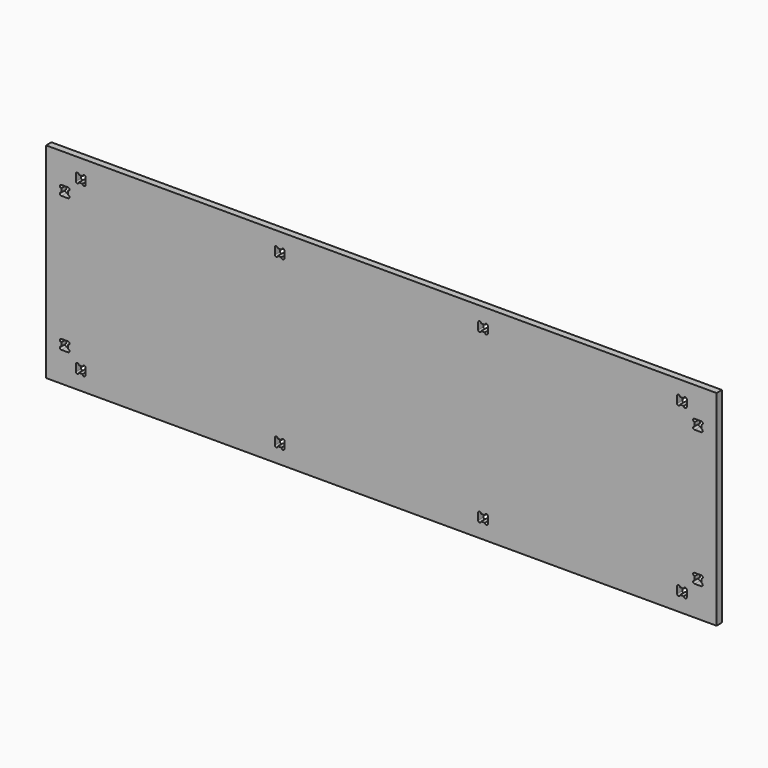
from build123d import *

# Parameters (mm, degrees)
F0_W     = 1800
F0_H     = 550
F1_DEPTH = 18


# Not quite as in the source:
# - ends of sketch curves that miss each other by under 0.0002 mm in the source are joined


with BuildPart() as f1:
    # F0 (on Front) → F1 (new body)
    with BuildSketch(Plane.XZ):
        Rectangle(F0_W, F0_H)
        with BuildLine():
            ThreePointArc((-812.0013296917, -234), (-816.0528989013, -237.9996675633), (-820, -233.8968701525))
            Line((-820, -233.8968701525), (-820, -216.0408403343))
            ThreePointArc((-820, -216.0408403343), (-816.0206289303, -212.0000521246), (-812.000208497, -216))
            Line((-812.000208497, -216), (-801.9986086037, -216))
            ThreePointArc((-801.9986086037, -216), (-797.945856423, -212.0003478642), (-794, -216.1054951861))
            Line((-794, -216.1054951861), (-794, -233.9987762793))
            Line((-794, -233.9987762793), (-794, -233.999999892))
            ThreePointArc((-794, -233.999999892), (-797.999999946, -237.9987762793), (-801.9999998128, -234))
            Line((-801.9999998128, -234), (-812.0013296917, -234))
        make_face(mode=Mode.SUBTRACT)
        with BuildLine():
            ThreePointArc((-859, -177.0002702016), (-862.9996675633, -172.948700992), (-858.8968701525, -169.0015998933))
            Line((-858.8968701525, -169.0015998933), (-841.0408403343, -169.0015998933))
            ThreePointArc((-841.0408403343, -169.0015998933), (-837.0000521246, -172.980970963), (-841, -177.0013913963))
            Line((-841, -177.0013913963), (-841, -187.0013913963))
            ThreePointArc((-841, -187.0013913963), (-837.0003478642, -191.054143577), (-841.1054951861, -195))
            Line((-841.1054951861, -195), (-858.8967770965, -195))
            ThreePointArc((-858.8967770965, -195), (-862.9996669629, -191.052947842), (-859, -187.0013320928))
            Line((-859, -187.0013320928), (-859, -177.0002702016))
        make_face(mode=Mode.SUBTRACT)
        with BuildLine():
            ThreePointArc((-278.0013430431, -234), (-282.0529122528, -237.9996675633), (-286.0000133514, -233.8968701525))
            Line((-286.0000133514, -233.8968701525), (-286.0000133514, -216.0408403343))
            ThreePointArc((-286.0000133514, -216.0408403343), (-282.0206422818, -212.0000521246), (-278.0002218485, -216))
            Line((-278.0002218485, -216), (-267.9986219552, -216))
            ThreePointArc((-267.9986219552, -216), (-263.9458697745, -212.0003478642), (-260.0000133514, -216.1054951861))
            Line((-260.0000133514, -216.1054951861), (-260.0000133514, -233.8967770965))
            ThreePointArc((-260.0000133514, -233.8967770965), (-263.9470655094, -237.9996669629), (-267.9986812587, -234))
            Line((-267.9986812587, -234), (-278.0013430431, -234))
        make_face(mode=Mode.SUBTRACT)
        with BuildLine():
            ThreePointArc((267.9986569569, -234), (263.9470877472, -237.9996675633), (259.9999866486, -233.8968701525))
            Line((259.9999866486, -233.8968701525), (259.9999866486, -216.0408403343))
            ThreePointArc((259.9999866486, -216.0408403343), (263.9793577182, -212.0000521246), (267.9997781515, -216))
            Line((267.9997781515, -216), (278.0027101376, -216))
            ThreePointArc((278.0027101376, -216), (282.002514573, -211.896777258), (285.9999866486, -216.0022722826))
            Line((285.9999866486, -216.0022722826), (285.9999866486, -233.793554193))
            ThreePointArc((285.9999866486, -233.793554193), (282.1045416448, -237.8954450037), (278.0026508341, -234))
            Line((278.0026508341, -234), (267.9986569569, -234))
        make_face(mode=Mode.SUBTRACT)
        with BuildLine():
            ThreePointArc((801.9986703083, -234), (797.9471010987, -237.9996675633), (794, -233.8968701525))
            Line((794, -233.8968701525), (794, -216.0408403343))
            ThreePointArc((794, -216.0408403343), (797.9793710697, -212.0000521246), (801.999791503, -216))
            Line((801.999791503, -216), (812.0013913963, -216))
            ThreePointArc((812.0013913963, -216), (816.054143577, -212.0003478642), (820, -216.1054951861))
            Line((820, -216.1054951861), (820, -233.8967770965))
            ThreePointArc((820, -233.8967770965), (816.052947842, -237.9996669629), (812.0013320928, -234))
            Line((812.0013320928, -234), (801.9986703083, -234))
        make_face(mode=Mode.SUBTRACT)
        with BuildLine():
            ThreePointArc((841, -177.0002702016), (837.0003324367, -172.948700992), (841.1031298475, -169.0015998933))
            Line((841.1031298475, -169.0015998933), (858.9591596657, -169.0015998933))
            ThreePointArc((858.9591596657, -169.0015998933), (862.9999478754, -172.980970963), (859, -177.0013913963))
            Line((859, -177.0013913963), (859, -187.0013913963))
            ThreePointArc((859, -187.0013913963), (862.9996521358, -191.054143577), (858.8945048139, -195))
            Line((858.8945048139, -195), (841.1032229035, -195))
            ThreePointArc((841.1032229035, -195), (837.0003330371, -191.052947842), (841, -187.0013320928))
            Line((841, -187.0013320928), (841, -177.0002702016))
        make_face(mode=Mode.SUBTRACT)
        with BuildLine():
            ThreePointArc((-859, 187.0013296917), (-862.9996675633, 191.0528989013), (-858.8968701525, 195))
            Line((-858.8968701525, 195), (-841.0408403343, 195))
            ThreePointArc((-841.0408403343, 195), (-837.0000521246, 191.0206289303), (-841, 187.000208497))
            Line((-841, 187.000208497), (-841, 176.9986086037))
            ThreePointArc((-841, 176.9986086037), (-837.0003478642, 172.945856423), (-841.1054951861, 169))
            Line((-841.1054951861, 169), (-858.8967770965, 169))
            ThreePointArc((-858.8967770965, 169), (-862.9996669629, 172.947052158), (-859, 176.9986679072))
            Line((-859, 176.9986679072), (-859, 187.0013296917))
        make_face(mode=Mode.SUBTRACT)
        with BuildLine():
            ThreePointArc((-812.0013296917, 216), (-816.0528989013, 212.0003324367), (-820, 216.1031298475))
            Line((-820, 216.1031298475), (-820, 233.9591596657))
            ThreePointArc((-820, 233.9591596657), (-816.0206289303, 237.9999478754), (-812.000208497, 234))
            Line((-812.000208497, 234), (-801.9986086037, 234))
            ThreePointArc((-801.9986086037, 234), (-797.945856423, 237.9996521358), (-794, 233.8945048139))
            Line((-794, 233.8945048139), (-794, 216.1032229035))
            ThreePointArc((-794, 216.1032229035), (-797.947052158, 212.0003330371), (-801.9986679072, 216))
            Line((-801.9986679072, 216), (-812.0013296917, 216))
        make_face(mode=Mode.SUBTRACT)
        with BuildLine():
            ThreePointArc((-278.0013296917, 216), (-282.0528989013, 212.0003324367), (-286, 216.1031298475))
            Line((-286, 216.1031298475), (-286, 233.9591596657))
            ThreePointArc((-286, 233.9591596657), (-282.0206289303, 237.9999478754), (-278.000208497, 234))
            Line((-278.000208497, 234), (-267.9986086037, 234))
            ThreePointArc((-267.9986086037, 234), (-263.945856423, 237.9996521358), (-260, 233.8945048139))
            Line((-260, 233.8945048139), (-260, 216.1032229035))
            ThreePointArc((-260, 216.1032229035), (-263.947052158, 212.0003330371), (-267.9986679072, 216))
            Line((-267.9986679072, 216), (-278.0013296917, 216))
        make_face(mode=Mode.SUBTRACT)
        with BuildLine():
            ThreePointArc((267.9986703083, 216), (263.9471010987, 212.0003324367), (260, 216.1031298475))
            Line((260, 216.1031298475), (260, 233.9591596657))
            ThreePointArc((260, 233.9591596657), (263.9793710697, 237.9999478754), (267.999791503, 234))
            Line((267.999791503, 234), (278.0013913963, 234))
            ThreePointArc((278.0013913963, 234), (282.054143577, 237.9996521358), (286, 233.8945048139))
            Line((286, 233.8945048139), (286, 216.1032229035))
            ThreePointArc((286, 216.1032229035), (282.052947842, 212.0003330371), (278.0013320928, 216))
            Line((278.0013320928, 216), (267.9986703083, 216))
        make_face(mode=Mode.SUBTRACT)
        with BuildLine():
            ThreePointArc((841, 187.0013296917), (837.0003324367, 191.0528989013), (841.1031298475, 195))
            Line((841.1031298475, 195), (858.9591596657, 195))
            ThreePointArc((858.9591596657, 195), (862.9999478754, 191.0206289303), (859, 187.000208497))
            Line((859, 187.000208497), (859, 176.9986086037))
            ThreePointArc((859, 176.9986086037), (862.9996521358, 172.945856423), (858.8945048139, 169))
            Line((858.8945048139, 169), (841.1032229035, 169))
            ThreePointArc((841.1032229035, 169), (837.0003330371, 172.947052158), (841, 176.9986679072))
            Line((841, 176.9986679072), (841, 187.0013296917))
        make_face(mode=Mode.SUBTRACT)
        with BuildLine():
            ThreePointArc((801.9986703083, 216), (797.9471010987, 212.0003324367), (794, 216.1031298475))
            Line((794, 216.1031298475), (794, 233.9591596657))
            ThreePointArc((794, 233.9591596657), (797.9793710697, 237.9999478754), (801.999791503, 234))
            Line((801.999791503, 234), (812.0013913963, 234))
            ThreePointArc((812.0013913963, 234), (816.054143577, 237.9996521358), (820, 233.8945048139))
            Line((820, 233.8945048139), (820, 216.1032229035))
            ThreePointArc((820, 216.1032229035), (816.052947842, 212.0003330371), (812.0013320928, 216))
            Line((812.0013320928, 216), (801.9986703083, 216))
        make_face(mode=Mode.SUBTRACT)
    extrude(amount=F1_DEPTH)


solid = f1.part
